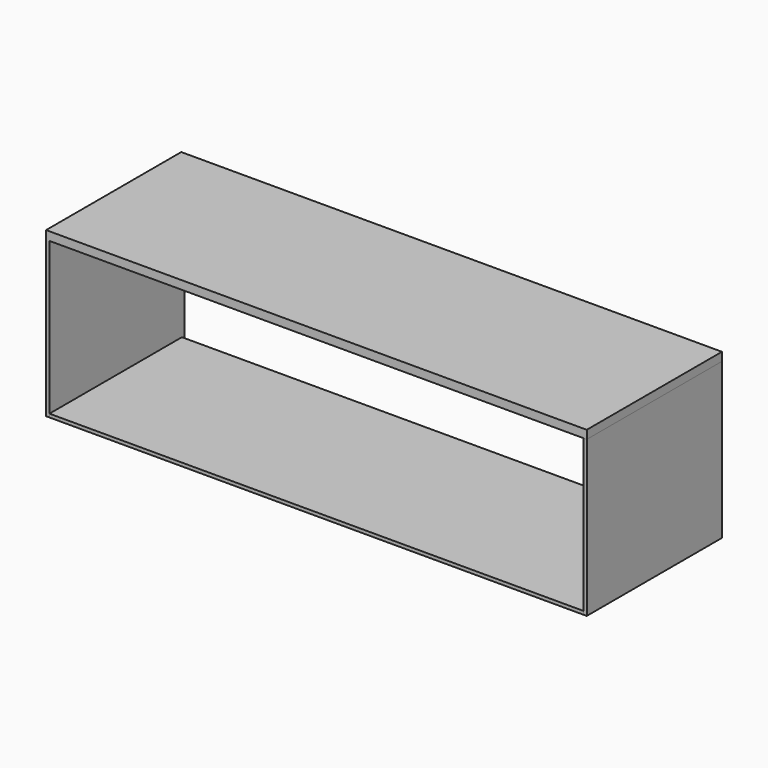
from build123d import *

# Parameters (mm, degrees)
F0_W     = 1600
F0_H     = 500
F1_DEPTH = 25
F3_W     = 1580
F3_H     = 490
F4_DEPTH = 10
F5_W     = 10
F5_H     = 500
F6_DEPTH = 460
F7_W     = 10
F7_H     = 500
F8_DEPTH = 460


with BuildPart() as f1:
    # F0 (on Top) → F1 (new body)
    with BuildSketch(Plane.XY):
        with Locations((800, 250)):
            Rectangle(F0_W, F0_H)
    extrude(amount=F1_DEPTH)

    # F5 (on face) → F6 (join, through all)
    with BuildSketch(Plane.XY):
        with Locations((5, 250)):
            Rectangle(F5_W, F5_H)
    extrude(amount=-F6_DEPTH)


with BuildPart() as f4:
    # F3 (on offset) → F4 (new body)
    with BuildSketch(Plane.XY.offset(-460)):
        with Locations((800, 245)):
            Rectangle(F3_W, F3_H)
    extrude(amount=F4_DEPTH)


with BuildPart() as f8:
    # F7 (on face) → F8 (new body, through all)
    with BuildSketch(Plane.XY):
        with Locations((1595, 250)):
            Rectangle(F7_W, F7_H)
    extrude(amount=-F8_DEPTH)


solid = Compound([f1.part, f4.part, f8.part])
